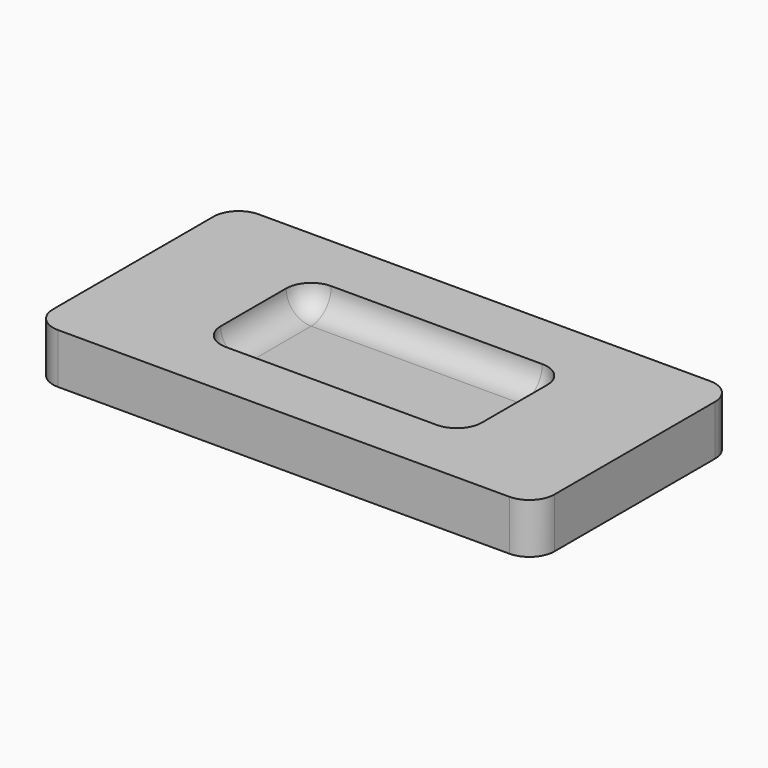
from build123d import *

# Parameters (mm, degrees)
F0_W     = 100
F0_H     = 50
F1_DEPTH = 10
F2_R     = 5
F3_W     = 52.0799309015
F3_H     = 26.2977816164
F4_DEPTH = 5
F5_R     = 5
F6_R     = 4.99999


# Not quite as in the source:
# - a fillet or chamfer is up to 0.001 mm smaller than in the source, because OpenCascade refuses the exact size


with BuildPart() as f1:
    # F0 (on Top) → F1 (new body)
    with BuildSketch(Plane.XY):
        Rectangle(F0_W, F0_H)
    extrude(amount=F1_DEPTH)

    # F2
    f2_edges = [f1.edges().sort_by_distance(p)[0] for p in [
        (-50, -25, 5),
        (-50, 25, 5),
        (50, -25, 5),
        (50, 25, 5),
    ]]
    fillet(f2_edges, radius=F2_R)

    # F3 (on face) → F4 (cut)
    with BuildSketch(Plane.XY.offset(10)):
        Rectangle(F3_W, F3_H)
    extrude(amount=-F4_DEPTH, mode=Mode.SUBTRACT)

    # F5
    f5_edges = [f1.edges().sort_by_distance(p)[0] for p in [
        (-26.039965, 13.148891, 7.5),
        (26.039965, 13.148891, 7.5),
        (26.039965, -13.148891, 7.5),
        (-26.039965, -13.148891, 7.5),
    ]]
    fillet(f5_edges, radius=F5_R)

    # F6 (radius 5 in the source; OpenCascade refuses exactly that, so slightly less here)
    f6_edges = [f1.edges().sort_by_distance(p)[0] for p in [
        (0, -13.148891, 5),
        (-24.575499, -11.684425, 5),
        (24.575499, -11.684425, 5),
        (-26.039965, 0, 5),
        (26.039965, 0, 5),
        (-24.575499, 11.684425, 5),
        (24.575499, 11.684425, 5),
        (0, 13.148891, 5),
    ]]
    fillet(f6_edges, radius=F6_R)


solid = f1.part
